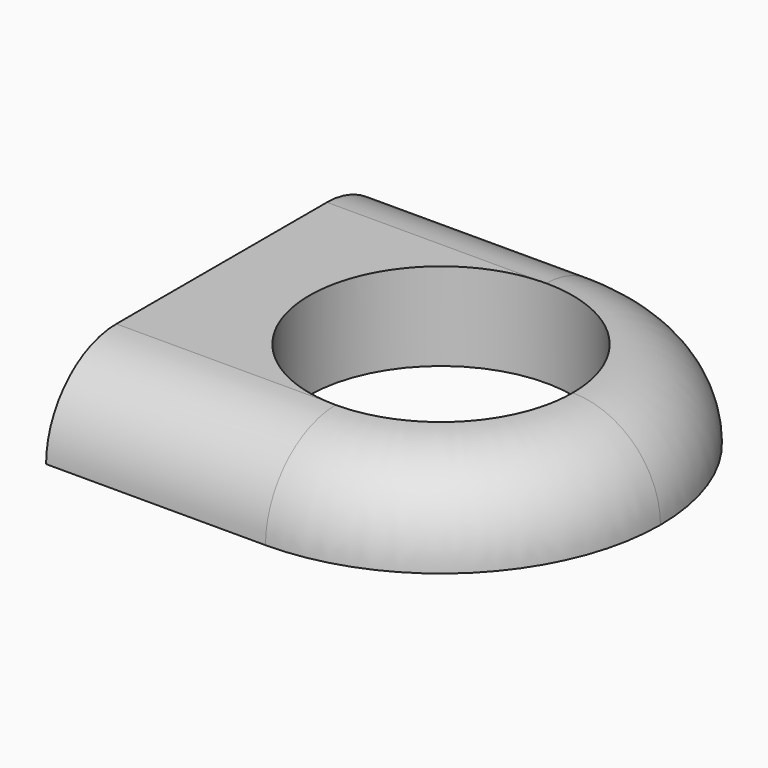
from build123d import *

# Parameters (mm, degrees)
F1_DEPTH = 2.54
F2_R     = 2.53999


# Not quite as in the source:
# - a fillet or chamfer is up to 0.001 mm smaller than in the source, because OpenCascade refuses the exact size


with BuildPart() as f1:
    # F0 (on Top) → F1 (new body)
    with BuildSketch(Plane.XY):
        with BuildLine():
            ThreePointArc((0, -6.35), (4.4901280605, -4.4901280605), (6.35, 0))
            ThreePointArc((6.35, 0), (4.4901280605, 4.4901280605), (0, 6.35))
            ThreePointArc((0, 6.35), (-4.4901280605, 4.4901280605), (-6.35, 0))
            ThreePointArc((-6.35, 0), (-4.4901280605, -4.4901280605), (0, -6.35))
        make_face()
        with BuildLine():
            ThreePointArc((3.81, 0), (0, -3.81), (-3.81, 0))
            ThreePointArc((-3.81, 0), (0, 3.81), (3.81, 0))
        make_face(mode=Mode.SUBTRACT)
        with BuildLine():
            ThreePointArc((-6.35, 0), (-4.4901280605, 4.4901280605), (0, 6.35))
            Line((0, 6.35), (-6.35, 6.35))
            Line((-6.35, 6.35), (-6.35, 0))
        make_face()
        with BuildLine():
            Line((-6.35, -6.35), (0, -6.35))
            ThreePointArc((0, -6.35), (-4.4901280605, -4.4901280605), (-6.35, 0))
            Line((-6.35, 0), (-6.35, -6.35))
        make_face()
    extrude(amount=F1_DEPTH)

    # F2 (radius 2.54 in the source; OpenCascade refuses exactly that, so slightly less here)
    f2_edges = [f1.edges().sort_by_distance(p)[0] for p in [
        (-3.175, 6.35, 2.54),
    ]]
    fillet(f2_edges, radius=F2_R)


solid = f1.part
